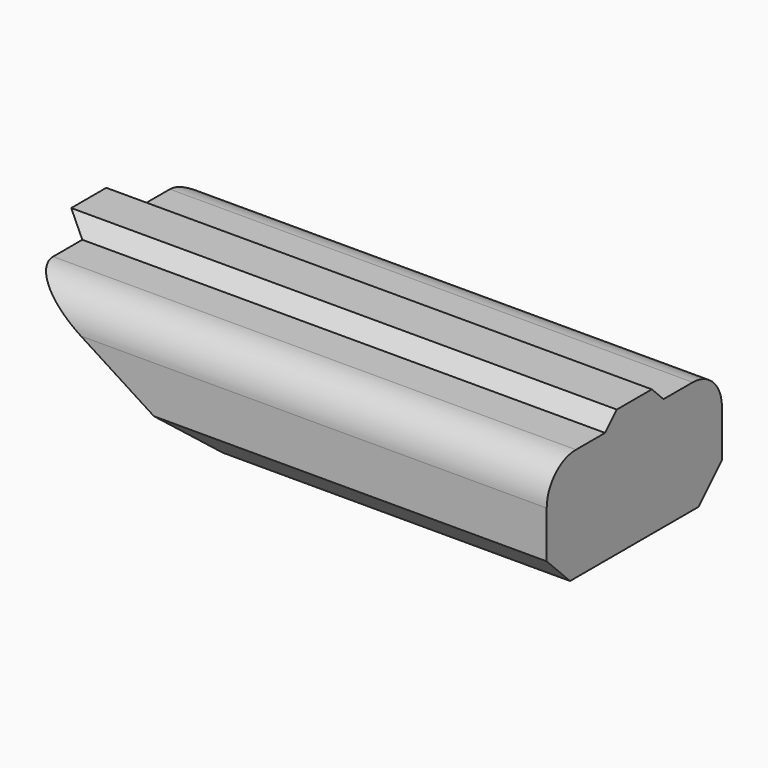
from build123d import *

# Parameters (mm, degrees)
F1_DEPTH    = 25.4
F2_SIZE     = 5.08
F3_SIZE     = 5.08
F4_DEPTH    = 25.4
F5_DEPTH    = 25.4
F6_SIZE     = 10.16
F7_SIZE     = 10.16
F9_T1_DEPTH = 245.4034453624
F10_T       = -2.54


# Not quite as in the source:
# - a fillet or chamfer that OpenCascade refuses, or shapes differently, is made with other operations: its cross-section is extruded or revolved along the edge and cut away or added
# - a feature of the source that left no trace in its solid (it failed there, or was rolled back) is left out


with BuildPart() as f1:
    # F0 (on Front) → F1 (new body)
    with BuildSketch(Plane.XZ):
        Polygon((65.9713447094, -32.0217311382), (65.9713447094, 12.2400075197), (-123.8519400358, 12.2400075197), (-54.8468492925, -32.0217311382), align=None)
    extrude(amount=F1_DEPTH)

    # F2
    f2_edges = [f1.edges().sort_by_distance(p)[0] for p in [
        (-28.940298, -25.4, 12.240008),
    ]]
    chamfer(f2_edges, length=F2_SIZE)

    # F3
    f3_edges = [f1.edges().sort_by_distance(p)[0] for p in [
        (-28.940298, 0, 12.240008),
    ]]
    chamfer(f3_edges, length=F3_SIZE)

    # F4 (add): a face of the model
    f4_faces = [f1.faces().sort_by_distance(p)[0] for p in [
        (-10.7362485924, 0, -11.1131350908),
    ]]
    extrude(f4_faces, amount=F4_DEPTH)

    # F5 (add): a face of the model
    f5_faces = [f1.faces().sort_by_distance(p)[0] for p in [
        (-10.7362485924, -25.4, -11.1131350908),
    ]]
    extrude(f5_faces, amount=F5_DEPTH)

    # F6
    f6_edges = [f1.edges().sort_by_distance(p)[0] for p in [
        (5.562248, 25.4, -32.021731),
    ]]
    chamfer(f6_edges, length=F6_SIZE)

    # F7
    f7_edges = [f1.edges().sort_by_distance(p)[0] for p in [
        (5.562248, -50.8, -32.021731),
    ]]
    chamfer(f7_edges, length=F7_SIZE)

    # F9: fillet of radius 12.7 on 4 edges, made by hand

    # F9_s2 → F9_t1 (cut)
    with BuildSketch(Plane.YZ.offset(-147.682100653)):
        with BuildLine():
            ThreePointArc((-50.8, -5.5399924803), (-47.0802561211, 3.4402636408), (-38.1, 7.1600075197))
            Line((-38.1, 7.1600075197), (-50.8, 7.1600075197))
            Line((-50.8, 7.1600075197), (-50.8, -5.5399924803))
        make_face()
        with BuildLine():
            ThreePointArc((25.4, -5.5399924803), (21.6802561211, 3.4402636408), (12.7, 7.1600075197))
            Line((12.7, 7.1600075197), (25.4, 7.1600075197))
            Line((25.4, 7.1600075197), (25.4, -5.5399924803))
        make_face()
    extrude(amount=F9_T1_DEPTH, mode=Mode.SUBTRACT)

    # F10
    f10_openings = [f1.faces().sort_by_distance(p)[0] for p in [
        (5.562248, -12.7, -32.021731),
    ]]
    offset(amount=F10_T, openings=f10_openings, kind=Kind.INTERSECTION)


solid = f1.part
